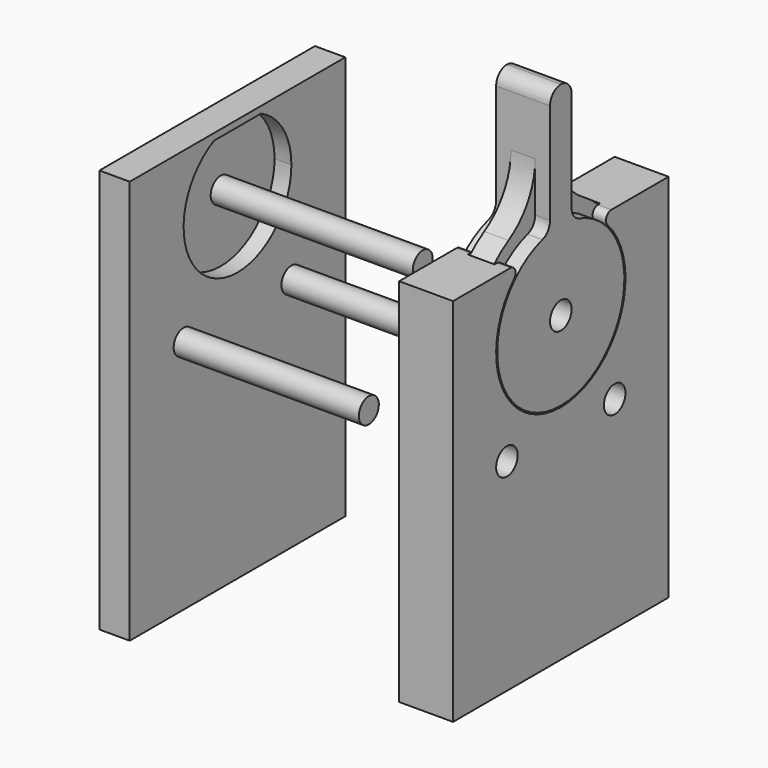
from build123d import *

# Parameters (mm, degrees)
F0_R      = 2.3495
F1_DEPTH  = 38.1
F2_W      = 50.8
F2_H      = 76.2
F3_DEPTH  = 2.54
F5_DEPTH  = 3.175
F6_R      = 2.3495
F7_DEPTH  = 34.925
F9_R      = 2.54
F10_DEPTH = 10.16
F11_R     = 1.27
F12_W     = 5.08
F12_H     = 9.2631512689
F14_W     = 2.54
F14_H     = 14.986
F16_R     = 2.54
F17_DEPTH = 10.16
F18_R     = 2.54
F19_DEPTH = 3.175
F21_W     = 10.16
F21_H     = 5.08
F22_DEPTH = 25.4
F23_R     = 2.54
F24_R     = 12.7
F25_R     = 2.53999


# Not quite as in the source:
# - a fillet or chamfer is up to 0.001 mm smaller than in the source, because OpenCascade refuses the exact size
# - a feature names something its author has since deleted; it is built from what else it names


with BuildPart() as f1:
    # F0 (on Right) → F1 (new body)
    with BuildSketch(Plane.YZ):
        Circle(F0_R)
    extrude(amount=F1_DEPTH)

    # F2 (on Right) → F3 (join)
    with BuildSketch(Plane.YZ):
        with Locations((0, -25.4)):
            Rectangle(F2_W, F2_H)
    extrude(amount=-F3_DEPTH)

    # F4 (on face) → F5 (join)
    with BuildSketch(Plane.YZ):
        Polygon((25.4, 12.7), (0, 12.7), (-25.4, 12.7), (-25.4, -63.5), (25.4, -63.5), align=None)
        with BuildLine():
            ThreePointArc((5.5358016583, 11.43), (10.7609172718, 6.7448246434), (12.7, 0))
            ThreePointArc((12.7, 0), (-6.7448246434, -10.7609172718), (-5.5358016583, 11.43))
            ThreePointArc((-5.5358016583, 11.43), (-2.8398063314, 12.3784288179), (0, 12.7))
            ThreePointArc((0, 12.7), (2.8398063314, 12.3784288179), (5.5358016583, 11.43))
        make_face(mode=Mode.SUBTRACT)
        with BuildLine():
            Line((-5.5358016583, 11.43), (5.5358016583, 11.43))
            ThreePointArc((5.5358016583, 11.43), (2.8398063314, 12.3784288179), (0, 12.7))
            ThreePointArc((0, 12.7), (-2.8398063314, 12.3784288179), (-5.5358016583, 11.43))
        make_face()
    extrude(amount=F5_DEPTH)

    # F6 (on face) → F7 (join, through all)
    with BuildSketch(Plane.YZ.offset(3.175)):
        with Locations((-12.7, -19.05)):
            Circle(F6_R)
        with Locations((12.7, -19.05)):
            Circle(F6_R)
    extrude(amount=F7_DEPTH)


with BuildPart() as f10:
    # F9 (on offset) → F10 (new body)
    with BuildSketch(Plane.YZ.offset(53.975)):
        with BuildLine():
            Line((-25.4, 12.7), (-25.4, -57.15))
            Line((-25.4, -57.15), (25.4, -57.15))
            Line((25.4, -57.15), (25.4, 12.7))
            Line((25.4, 12.7), (8.4242269675, 12.7))
            ThreePointArc((8.4242269675, 12.7), (13.4283807472, 7.2066768006), (15.24, 0))
            ThreePointArc((15.24, 0), (-7.2066768006, -13.4283807472), (-8.4242269675, 12.7))
            Line((-8.4242269675, 12.7), (-25.4, 12.7))
        make_face()
        with Locations((-12.7, -19.05)):
            Circle(F9_R, mode=Mode.SUBTRACT)
        with Locations((12.7, -19.05)):
            Circle(F9_R, mode=Mode.SUBTRACT)
    extrude(amount=F10_DEPTH)

    # F11
    f11_edges = [f10.edges().sort_by_distance(p)[0] for p in [
        (59.055, 8.424227, 12.7),
        (59.055, -8.424227, 12.7),
    ]]
    fillet(f11_edges, radius=F11_R)

    # F12 (on Top) → F13 (revolve, cut)
    with BuildSketch(Plane.XY):
        with Locations((59.055, 13.1484243655)):
            Rectangle(F12_W, F12_H)
    revolve(axis=Axis((28.3873360604, 0, 0), (1, 0, 0)), mode=Mode.SUBTRACT)


with BuildPart() as f15:
    # F14 (on Top) → F15 (revolve)
    with BuildSketch(Plane.XY):
        with Locations((55.245, 7.493)):
            Rectangle(F14_W, F14_H)
        Polygon((56.769, 14.986), (56.515, 14.986), (56.515, 0), (61.595, 0), (61.595, 14.986), (61.341, 14.986), (61.341, 17.526), (56.769, 17.526), align=None)
        with Locations((62.865, 7.493)):
            Rectangle(F14_W, F14_H)
    revolve(axis=Axis((59.055, 0, 0), (1, 0, 0)))

    # F16 (on face) → F17 (cut, through all)
    with BuildSketch(Plane.YZ.offset(64.135)):
        Circle(F16_R)
    extrude(amount=-F17_DEPTH, mode=Mode.SUBTRACT)

    # F18 (on face) → F19 (cut)
    with BuildSketch(Plane(origin=(53.975, 0, 0), x_dir=(0, -1, 0), z_dir=(-1, 0, 0))):
        with BuildLine():
            ThreePointArc((0, 12.7), (-8.9802561211, -8.9802561211), (12.7, 0))
            ThreePointArc((12.7, 0), (11.9966334008, 4.1678276171), (9.9644429849, 7.874))
            Line((9.9644429849, 7.874), (0, 12.7))
        make_face()
        Circle(F18_R, mode=Mode.SUBTRACT)
    extrude(amount=-F19_DEPTH, mode=Mode.SUBTRACT)

    # F21 (on offset) → F22 (join)
    with BuildSketch(Plane.XY.offset(12.954)):
        with Locations((59.055, 0)):
            Rectangle(F21_W, F21_H)
    extrude(amount=F22_DEPTH)

    # F23
    f23_edges = [f15.edges().sort_by_distance(p)[0] for p in [
        (62.738, -2.54, 14.769177),
        (62.738, 2.54, 14.769177),
        (55.372, -2.54, 14.769177),
        (55.372, 2.54, 14.769177),
    ]]
    fillet(f23_edges, radius=F23_R)

    # F24
    f24_edges = [f15.edges().sort_by_distance(p)[0] for p in [
        (59.055, 2.54, 17.340965),
        (59.055, -2.54, 17.340965),
    ]]
    fillet(f24_edges, radius=F24_R)

    # F25 (radius 2.54 in the source; OpenCascade refuses exactly that, so slightly less here)
    f25_edges = [f15.edges().sort_by_distance(p)[0] for p in [
        (59.055, -2.54, 38.354),
        (59.055, 2.54, 38.354),
    ]]
    fillet(f25_edges, radius=F25_R)


solid = Compound([f1.part, f10.part, f15.part])
